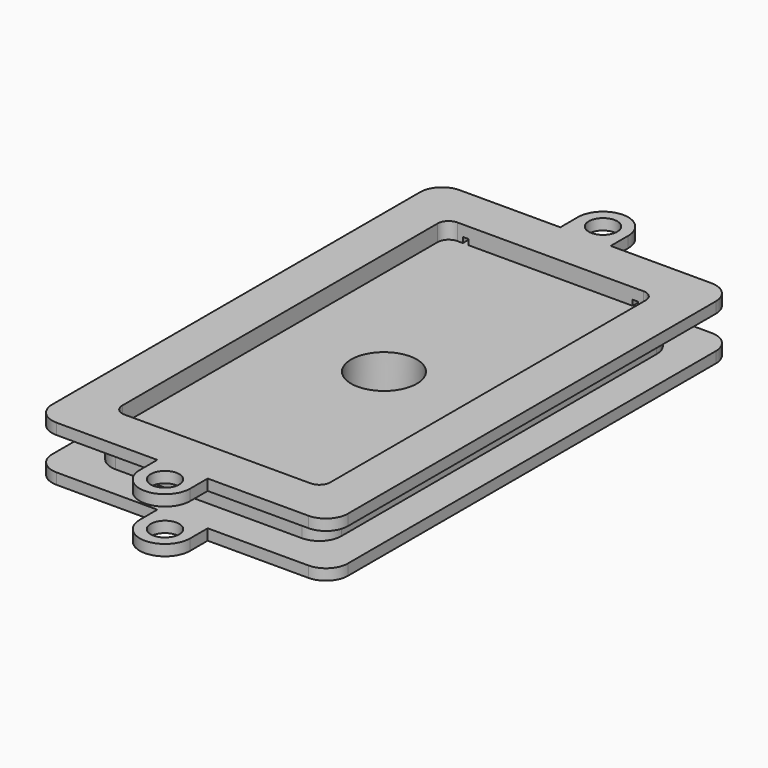
from build123d import *

# Parameters (mm, degrees)
F1_DEPTH  = 1
F3_DEPTH  = 3
F4_DEPTH  = 1.001
F6_DEPTH  = 1
F7_R      = 1.3
F8_DEPTH  = 1
F10_W     = 19
F10_H     = 38
F11_DEPTH = 1
F12_R     = 3
F13_DEPTH = 25
F14_R     = 5
F14_R_2   = 3
F15_DEPTH = 2.5
F16_W     = 0.5
F16_H     = 0.5
F17_DEPTH = 5


# Not quite as in the source:
# - a pattern or mirror of a feature is missing from the dataset's text; its kind, count and spacing are read off the source's solid


with BuildPart() as f1:
    # F0 (on Top) → F1 (new body)
    with BuildSketch(Plane.XY):
        with BuildLine():
            ThreePointArc((13.5, 21), (12.9142135624, 22.4142135624), (11.5, 23))
            Line((11.5, 23), (-11.5, 23))
            ThreePointArc((-11.5, 23), (-12.9142135624, 22.4142135624), (-13.5, 21))
            Line((-13.5, 21), (-13.5, -21))
            ThreePointArc((-13.5, -21), (-12.9142135624, -22.4142135624), (-11.5, -23))
            Line((-11.5, -23), (11.5, -23))
            ThreePointArc((11.5, -23), (12.9142135624, -22.4142135624), (13.5, -21))
            Line((13.5, -21), (13.5, 21))
        make_face()
    extrude(amount=F1_DEPTH)

    # F2 (on face) → F3 (join)
    with BuildSketch(Plane.XY.offset(1)):
        with BuildLine():
            ThreePointArc((10.5, 18), (9.9142135624, 19.4142135624), (8.5, 20))
            Line((8.5, 20), (-8.5, 20))
            ThreePointArc((-8.5, 20), (-9.9142135624, 19.4142135624), (-10.5, 18))
            Line((-10.5, 18), (-10.5, -18))
            ThreePointArc((-10.5, -18), (-9.9142135624, -19.4142135624), (-8.5, -20))
            Line((-8.5, -20), (8.5, -20))
            ThreePointArc((8.5, -20), (9.9142135624, -19.4142135624), (10.5, -18))
            Line((10.5, -18), (10.5, 18))
        make_face()
        with BuildLine():
            ThreePointArc((8.5, 19), (9.2071067812, 18.7071067812), (9.5, 18))
            Line((9.5, 18), (9.5, -18))
            ThreePointArc((9.5, -18), (9.2071067812, -18.7071067812), (8.5, -19))
            Line((8.5, -19), (-8.5, -19))
            ThreePointArc((-8.5, -19), (-9.2071067812, -18.7071067812), (-9.5, -18))
            Line((-9.5, -18), (-9.5, 18))
            ThreePointArc((-9.5, 18), (-9.2071067812, 18.7071067812), (-8.5, 19))
            Line((-8.5, 19), (8.5, 19))
        make_face(mode=Mode.SUBTRACT)
    extrude(amount=F3_DEPTH)

    # F4 (cut, through all): a face of the model
    f4_faces = [f1.faces().sort_by_distance(p)[0] for p in [
        (0, 0, 1),
    ]]
    extrude(f4_faces, amount=-F4_DEPTH, mode=Mode.SUBTRACT)

    # F5 (on face) → F6 (join)
    with BuildSketch(Plane.XY.offset(4)):
        with BuildLine():
            Line((13.5, -21), (13.5, 21))
            ThreePointArc((13.5, 21), (12.9142135624, 22.4142135624), (11.5, 23))
            Line((11.5, 23), (-11.5, 23))
            ThreePointArc((-11.5, 23), (-12.9142135624, 22.4142135624), (-13.5, 21))
            Line((-13.5, 21), (-13.5, -21))
            ThreePointArc((-13.5, -21), (-12.9142135624, -22.4142135624), (-11.5, -23))
            Line((-11.5, -23), (11.5, -23))
            ThreePointArc((11.5, -23), (12.9142135624, -22.4142135624), (13.5, -21))
        make_face()
        with BuildLine():
            ThreePointArc((8.5, 19), (9.2071067812, 18.7071067812), (9.5, 18))
            Line((9.5, 18), (9.5, -18))
            ThreePointArc((9.5, -18), (9.2071067812, -18.7071067812), (8.5, -19))
            Line((8.5, -19), (-8.5, -19))
            ThreePointArc((-8.5, -19), (-9.2071067812, -18.7071067812), (-9.5, -18))
            Line((-9.5, -18), (-9.5, 18))
            ThreePointArc((-9.5, 18), (-9.2071067812, 18.7071067812), (-8.5, 19))
            Line((-8.5, 19), (8.5, 19))
        make_face(mode=Mode.SUBTRACT)
    extrude(amount=F6_DEPTH)

    # F7 (on Top) → F8 (join)
    with BuildSketch(Plane.XY):
        with BuildLine():
            Line((2.3, 23), (2.3, 25))
            ThreePointArc((2.3, 25), (0, 27.3), (-2.3, 25))
            Line((-2.3, 25), (-2.3, 23))
            Line((-2.3, 23), (2.3, 23))
        make_face()
        with Locations((0, 25)):
            Circle(F7_R, mode=Mode.SUBTRACT)
        with BuildLine():
            ThreePointArc((-2.3, -25), (0, -27.3), (2.3, -25))
            Line((2.3, -25), (2.3, -23))
            Line((2.3, -23), (-2.3, -23))
            Line((-2.3, -23), (-2.3, -25))
        make_face()
        with Locations((0, -25)):
            Circle(F7_R, mode=Mode.SUBTRACT)
    f8 = extrude(amount=F8_DEPTH)

    # F8_copies: F8 across plane
    add(f8.mirror(Plane.XY.offset(2.5)))

    # F10 (on mid) → F11 (join)
    with BuildSketch(Plane(origin=(0, 0, 2.5), x_dir=(1, 0, 0), z_dir=(0, 0, -1))):
        Rectangle(F10_W, F10_H)
    extrude(amount=-F11_DEPTH)

    # F12 (on face) → F13 (cut)
    with BuildSketch(Plane.XY.offset(3.5)):
        Circle(F12_R)
    extrude(amount=-F13_DEPTH, mode=Mode.SUBTRACT)

    # F14 (on face) → F15 (join, through all)
    with BuildSketch(Plane(origin=(0, 0, 2.5), x_dir=(1, 0, 0), z_dir=(0, 0, -1))):
        Circle(F14_R)
        Circle(F14_R_2, mode=Mode.SUBTRACT)
    extrude(amount=F15_DEPTH)

    # F16 (on face) → F17 (cut)
    with BuildSketch(Plane(origin=(0, 20, 0), x_dir=(-1, 0, 0), z_dir=(0, 1, 0))):
        with Locations((-7.75, 3.75)):
            Rectangle(F16_W, F16_H)
        with Locations((7.75, 3.75)):
            Rectangle(F16_W, F16_H)
    extrude(amount=-F17_DEPTH, mode=Mode.SUBTRACT)


solid = f1.part
